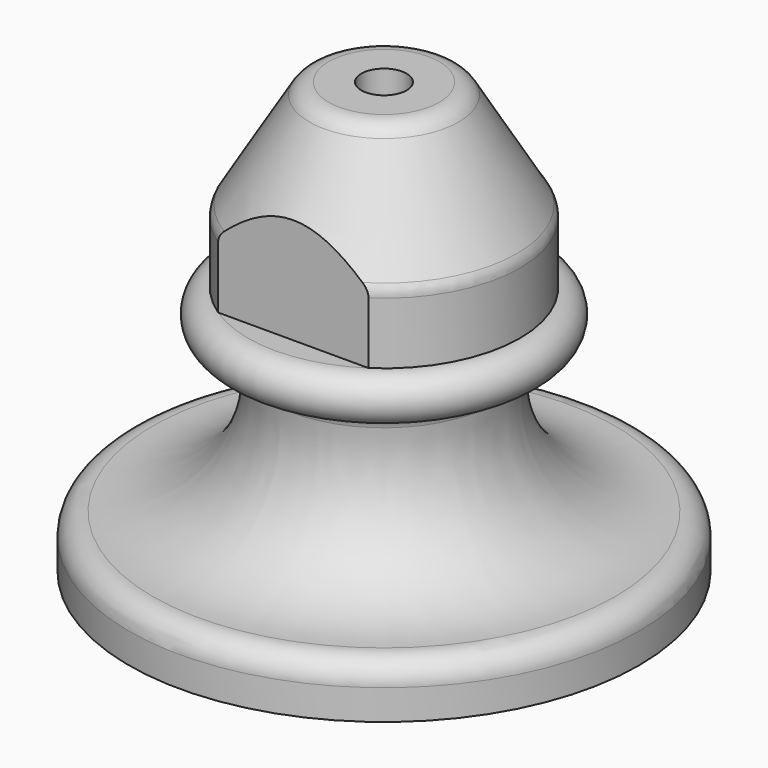
from build123d import *

# Parameters (mm, degrees)
F2_W          = 9.1512240469
F2_H          = 19.1432087421
F2_W_2        = 12.2216980672
F2_H_2        = 16.8554036617
F3_DEPTH      = 25
F3_DEPTH_BACK = 25


# Not quite as in the source:
# - a feature names something its author has since deleted; it is built from what else it names


with BuildPart() as f1:
    # F0 (on Front) → F1 (revolve)
    with BuildSketch(Plane.XZ):
        with BuildLine():
            Line((4.8676192421, 38), (2, 38))
            Line((2, 38), (2, 25))
            Line((2, 25), (5, 25))
            ThreePointArc((5, 25), (6.4142135624, 24.4142135624), (7, 23))
            Line((7, 23), (7, 12.7096224699))
            ThreePointArc((7, 12.7096224699), (10.6247219646, 5.4898848922), (17.8140384111, 1.8051937189))
            ThreePointArc((17.8140384111, 1.8051937189), (18.9645863819, 1.1919815957), (19.492762126, 0))
            Line((19.492762126, 0), (19.5, 0))
            Line((19.5, 0), (22.5, 0))
            Line((22.5, 0), (22.5, 2.6612672701))
            ThreePointArc((22.5, 2.6612672701), (21.8756991001, 4.1129738472), (20.3925480139, 4.6583787018))
            ThreePointArc((20.3925480139, 4.6583787018), (12.3842952255, 7.9968112401), (10, 16.3390160333))
            ThreePointArc((10, 16.3390160333), (10.6822659141, 17.5293841713), (11.9710575281, 17.9999999987))
            Line((11.9710575281, 17.9999999987), (12, 18))
            ThreePointArc((12, 18), (13.9999999114, 20), (12, 22))
            Line((12, 22), (12, 27.4460320701))
            ThreePointArc((12, 27.4460320701), (11.9274298564, 27.9798992339), (11.7149858514, 28.475023581))
            Line((11.7149858514, 28.475023581), (6.5826050935, 37.0289915109))
            ThreePointArc((6.5826050935, 37.0289915109), (5.853016872, 37.7403998135), (4.8676192421, 38))
        make_face()
    revolve(axis=Axis((0, 0, 19), (0, 0, -1)))

    # F2 (on Right) → F3 (cut, two sides)
    with BuildSketch(Plane.YZ) as f3_sk:
        with Locations((14.5756120235, 31.5716043711)):
            Rectangle(F2_W, F2_H)
        with Locations((-16.1108490336, 30.4277018309)):
            Rectangle(F2_W_2, F2_H_2)
    extrude(amount=-F3_DEPTH, mode=Mode.SUBTRACT)
    extrude(f3_sk.sketch, amount=F3_DEPTH_BACK, mode=Mode.SUBTRACT)


solid = f1.part
